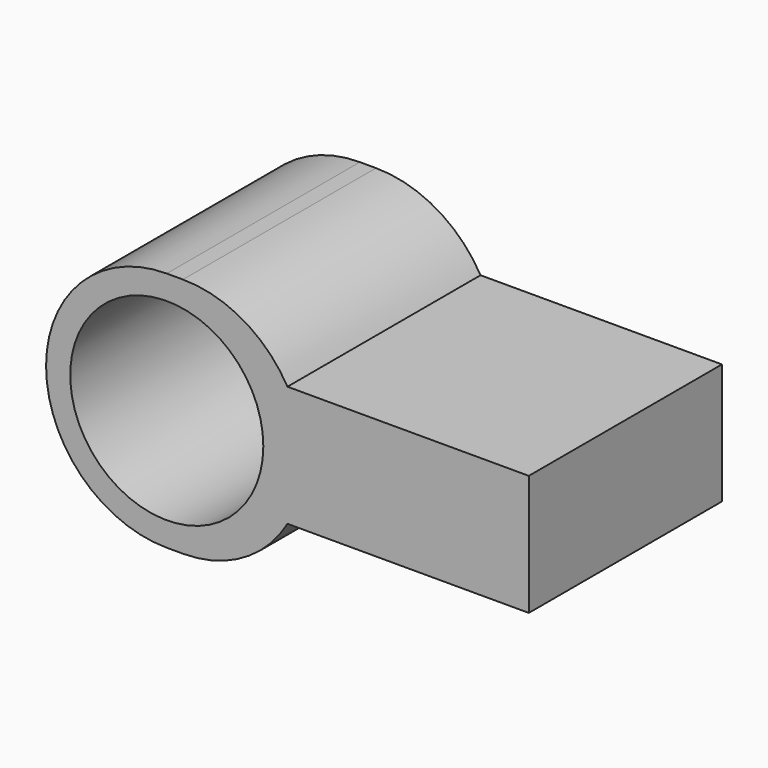
from build123d import *

# Parameters (mm, degrees)
F0_R        = 10.16
F1_DEPTH    = 25.4
F2_T1_DEPTH = 80.3926131403
F2_T3_DEPTH = 88.9


# Not quite as in the source:
# - a fillet or chamfer that OpenCascade refuses, or shapes differently, is made with other operations: its cross-section is extruded or revolved along the edge and cut away or added


with BuildPart() as f1:
    # F0 (on Front) → F1 (new body)
    with BuildSketch(Plane.XZ):
        Polygon((-13.2853005409, 12.7), (-38.6853005409, 12.7), (-38.6853005409, -12.7), (-13.2853005409, -12.7), (-13.2853005409, -6.35), (12.1146994591, -6.35), (12.1146994591, 6.35), (-13.2853005409, 6.35), align=None)
        with Locations((-25.9853005409, 0)):
            Circle(F0_R, mode=Mode.SUBTRACT)
    extrude(amount=F1_DEPTH)

    # F2: fillet of radius 12.7 on 4 edges, made by hand

    # F2_s2 → F2_t1 (cut)
    with BuildSketch(Plane.XZ.offset(-27.4963065702)):
        with BuildLine():
            ThreePointArc((-13.2853005409, 6.35), (-17.933823169, 10.9985226281), (-24.283823169, 12.7))
            Line((-24.283823169, 12.7), (-13.2853005409, 12.7))
            Line((-13.2853005409, 12.7), (-13.2853005409, 6.35))
        make_face()
        with BuildLine():
            ThreePointArc((-24.283823169, -12.7), (-17.933823169, -10.9985226281), (-13.2853005409, -6.35))
            Line((-13.2853005409, -6.35), (-13.2853005409, -12.7))
            Line((-13.2853005409, -12.7), (-24.283823169, -12.7))
        make_face()
    extrude(amount=F2_T1_DEPTH, mode=Mode.SUBTRACT)

    # F2_s4 → F2_t3 (cut)
    with BuildSketch(Plane.XZ.offset(-31.75)):
        with BuildLine():
            ThreePointArc((-25.9853005409, 12.7), (-34.965556662, 8.9802561211), (-38.6853005409, 0))
            Line((-38.6853005409, 0), (-38.6853005409, 12.7))
            Line((-38.6853005409, 12.7), (-25.9853005409, 12.7))
        make_face()
        with BuildLine():
            ThreePointArc((-38.6853005409, 0), (-34.965556662, -8.9802561211), (-25.9853005409, -12.7))
            Line((-25.9853005409, -12.7), (-38.6853005409, -12.7))
            Line((-38.6853005409, -12.7), (-38.6853005409, 0))
        make_face()
    extrude(amount=F2_T3_DEPTH, mode=Mode.SUBTRACT)


solid = f1.part
